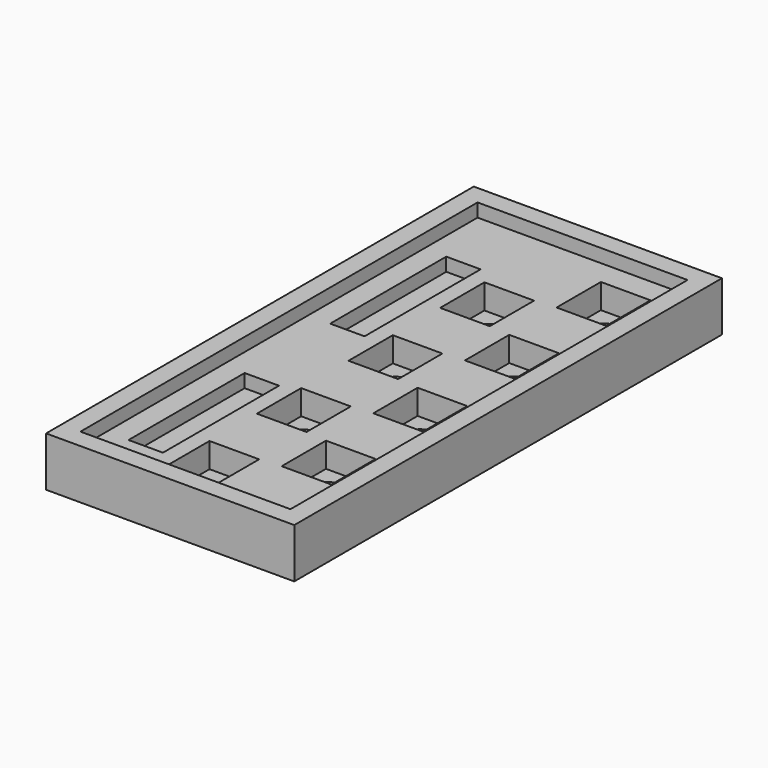
from build123d import *

# Parameters (mm, degrees)
F0_W     = 65
F0_H     = 140
F0_W_2   = 9
F0_H_2   = 38
F0_W_3   = 13
F0_H_3   = 14.5
F0_R     = 3.85
F1_DEPTH = 3
F2_DEPTH = 6
F3_DEPTH = 9.5
F4_DEPTH = 13


# Not quite as in the source:
# - a feature names something its author has since deleted; it is built from what else it names


with BuildPart() as f1:
    # F0 (on Top) → F1 (new body)
    with BuildSketch(Plane.XY):
        with Locations((-31.25, -0.0599437952)):
            Rectangle(F0_W, F0_H)
        Polygon((-58.75, -65.0599437952), (-58.75, 64.9400562048), (-3.75, 64.9400562048), (-3.75, 60.4400562048), (-3.75, 49.5400562048), (-3.75, -65.0599437952), align=None, mode=Mode.SUBTRACT)
        Polygon((-3.75, 64.9400562048), (-58.75, 64.9400562048), (-58.75, -65.0599437952), (-3.75, -65.0599437952), (-3.75, 49.5400562048), (-3.75, 60.4400562048), align=None)
        with Locations((-48.45, -37.5599437952)):
            Rectangle(F0_W_2, F0_H_2, mode=Mode.SUBTRACT)
        with Locations((-33.25, -53.8099437952)):
            Rectangle(F0_W_3, F0_H_3, mode=Mode.SUBTRACT)
        with Locations((-33.25, -23.8099437952)):
            Rectangle(F0_W_3, F0_H_3, mode=Mode.SUBTRACT)
        with Locations((-14.75, -38.8099437952)):
            Rectangle(F0_W_3, F0_H_3, mode=Mode.SUBTRACT)
        with Locations((-14.75, -8.8099437952)):
            Rectangle(F0_W_3, F0_H_3, mode=Mode.SUBTRACT)
        with Locations((-48.45, 28.4400562048)):
            Rectangle(F0_W_2, F0_H_2, mode=Mode.SUBTRACT)
        with Locations((-33.25, 6.1900562048)):
            Rectangle(F0_W_3, F0_H_3, mode=Mode.SUBTRACT)
        with Locations((-33.25, 36.1900562048)):
            Rectangle(F0_W_3, F0_H_3, mode=Mode.SUBTRACT)
        with Locations((-14.75, 21.1900562048)):
            Rectangle(F0_W_3, F0_H_3, mode=Mode.SUBTRACT)
        with Locations((-14.75, 51.1900562048)):
            Rectangle(F0_W_3, F0_H_3, mode=Mode.SUBTRACT)
        with Locations((-48.45, 28.4400562048)):
            Rectangle(F0_W_2, F0_H_2)
        with Locations((-48.45, -37.5599437952)):
            Rectangle(F0_W_2, F0_H_2)
        with Locations((-14.75, 51.1900562048)):
            Rectangle(F0_W_3, F0_H_3)
        with Locations((-14.75, 51.1900562048)):
            Circle(F0_R, mode=Mode.SUBTRACT)
        with Locations((-33.25, 36.1900562048)):
            Rectangle(F0_W_3, F0_H_3)
        with Locations((-33.25, 36.1900562048)):
            Circle(F0_R, mode=Mode.SUBTRACT)
        with Locations((-14.75, 21.1900562048)):
            Rectangle(F0_W_3, F0_H_3)
        with Locations((-14.75, 21.1900562048)):
            Circle(F0_R, mode=Mode.SUBTRACT)
        with Locations((-33.25, 6.1900562048)):
            Rectangle(F0_W_3, F0_H_3)
        with Locations((-33.25, 6.1900562048)):
            Circle(F0_R, mode=Mode.SUBTRACT)
        with Locations((-14.75, -8.8099437952)):
            Rectangle(F0_W_3, F0_H_3)
        with Locations((-14.75, -8.8099437952)):
            Circle(F0_R, mode=Mode.SUBTRACT)
        with Locations((-33.25, -23.8099437952)):
            Rectangle(F0_W_3, F0_H_3)
        with Locations((-33.25, -23.8099437952)):
            Circle(F0_R, mode=Mode.SUBTRACT)
        with Locations((-33.25, -53.8099437952)):
            Rectangle(F0_W_3, F0_H_3)
        with Locations((-33.25, -53.8099437952)):
            Circle(F0_R, mode=Mode.SUBTRACT)
        with Locations((-14.75, -38.8099437952)):
            Rectangle(F0_W_3, F0_H_3)
        with Locations((-14.75, -38.8099437952)):
            Circle(F0_R, mode=Mode.SUBTRACT)
    extrude(amount=F1_DEPTH)

    # F0 (on Top) → F2 (join)
    with BuildSketch(Plane.XY):
        with Locations((-31.25, -0.0599437952)):
            Rectangle(F0_W, F0_H)
        Polygon((-58.75, -65.0599437952), (-58.75, 64.9400562048), (-3.75, 64.9400562048), (-3.75, 60.4400562048), (-3.75, 49.5400562048), (-3.75, -65.0599437952), align=None, mode=Mode.SUBTRACT)
        Polygon((-3.75, 64.9400562048), (-58.75, 64.9400562048), (-58.75, -65.0599437952), (-3.75, -65.0599437952), (-3.75, 49.5400562048), (-3.75, 60.4400562048), align=None)
        with Locations((-48.45, -37.5599437952)):
            Rectangle(F0_W_2, F0_H_2, mode=Mode.SUBTRACT)
        with Locations((-33.25, -53.8099437952)):
            Rectangle(F0_W_3, F0_H_3, mode=Mode.SUBTRACT)
        with Locations((-33.25, -23.8099437952)):
            Rectangle(F0_W_3, F0_H_3, mode=Mode.SUBTRACT)
        with Locations((-14.75, -38.8099437952)):
            Rectangle(F0_W_3, F0_H_3, mode=Mode.SUBTRACT)
        with Locations((-14.75, -8.8099437952)):
            Rectangle(F0_W_3, F0_H_3, mode=Mode.SUBTRACT)
        with Locations((-48.45, 28.4400562048)):
            Rectangle(F0_W_2, F0_H_2, mode=Mode.SUBTRACT)
        with Locations((-33.25, 6.1900562048)):
            Rectangle(F0_W_3, F0_H_3, mode=Mode.SUBTRACT)
        with Locations((-33.25, 36.1900562048)):
            Rectangle(F0_W_3, F0_H_3, mode=Mode.SUBTRACT)
        with Locations((-14.75, 21.1900562048)):
            Rectangle(F0_W_3, F0_H_3, mode=Mode.SUBTRACT)
        with Locations((-14.75, 51.1900562048)):
            Rectangle(F0_W_3, F0_H_3, mode=Mode.SUBTRACT)
        with Locations((-48.45, 28.4400562048)):
            Rectangle(F0_W_2, F0_H_2)
        with Locations((-48.45, -37.5599437952)):
            Rectangle(F0_W_2, F0_H_2)
    extrude(amount=F2_DEPTH)

    # F0 (on Top) → F3 (join)
    with BuildSketch(Plane.XY):
        with Locations((-31.25, -0.0599437952)):
            Rectangle(F0_W, F0_H)
        Polygon((-58.75, -65.0599437952), (-58.75, 64.9400562048), (-3.75, 64.9400562048), (-3.75, 60.4400562048), (-3.75, 49.5400562048), (-3.75, -65.0599437952), align=None, mode=Mode.SUBTRACT)
        Polygon((-3.75, 64.9400562048), (-58.75, 64.9400562048), (-58.75, -65.0599437952), (-3.75, -65.0599437952), (-3.75, 49.5400562048), (-3.75, 60.4400562048), align=None)
        with Locations((-48.45, -37.5599437952)):
            Rectangle(F0_W_2, F0_H_2, mode=Mode.SUBTRACT)
        with Locations((-33.25, -53.8099437952)):
            Rectangle(F0_W_3, F0_H_3, mode=Mode.SUBTRACT)
        with Locations((-33.25, -23.8099437952)):
            Rectangle(F0_W_3, F0_H_3, mode=Mode.SUBTRACT)
        with Locations((-14.75, -38.8099437952)):
            Rectangle(F0_W_3, F0_H_3, mode=Mode.SUBTRACT)
        with Locations((-14.75, -8.8099437952)):
            Rectangle(F0_W_3, F0_H_3, mode=Mode.SUBTRACT)
        with Locations((-48.45, 28.4400562048)):
            Rectangle(F0_W_2, F0_H_2, mode=Mode.SUBTRACT)
        with Locations((-33.25, 6.1900562048)):
            Rectangle(F0_W_3, F0_H_3, mode=Mode.SUBTRACT)
        with Locations((-33.25, 36.1900562048)):
            Rectangle(F0_W_3, F0_H_3, mode=Mode.SUBTRACT)
        with Locations((-14.75, 21.1900562048)):
            Rectangle(F0_W_3, F0_H_3, mode=Mode.SUBTRACT)
        with Locations((-14.75, 51.1900562048)):
            Rectangle(F0_W_3, F0_H_3, mode=Mode.SUBTRACT)
    extrude(amount=F3_DEPTH)

    # F0 (on Top) → F4 (join)
    with BuildSketch(Plane.XY):
        with Locations((-31.25, -0.0599437952)):
            Rectangle(F0_W, F0_H)
        Polygon((-58.75, -65.0599437952), (-58.75, 64.9400562048), (-3.75, 64.9400562048), (-3.75, 60.4400562048), (-3.75, 49.5400562048), (-3.75, -65.0599437952), align=None, mode=Mode.SUBTRACT)
    extrude(amount=F4_DEPTH)


solid = f1.part
